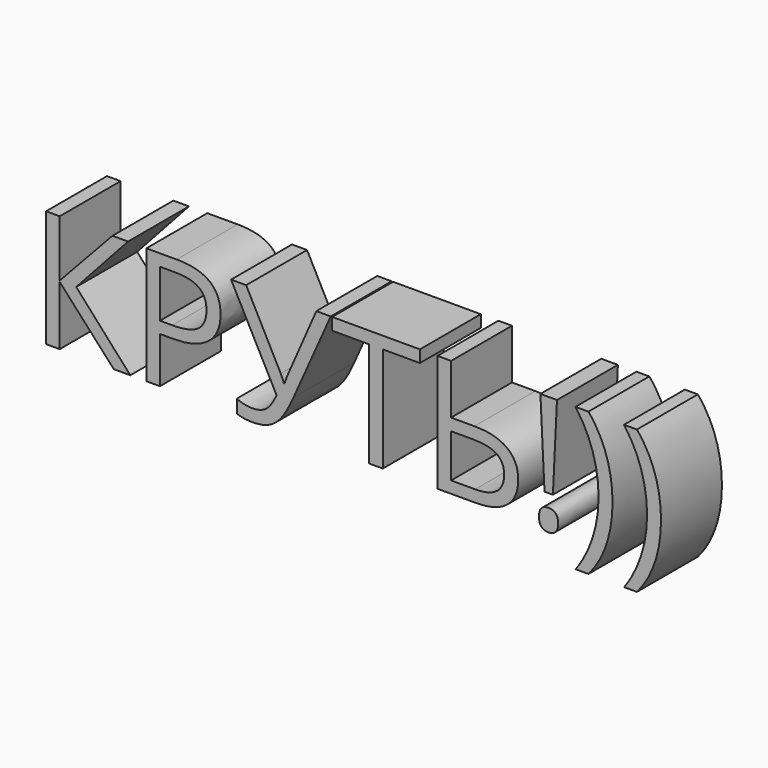
from build123d import *

# Parameters (mm, degrees)
F0_TEXT_SIZE = 53.8159886168
F1_DEPTH     = 25


# Not quite as in the source:
# - Text() gives the source's letters only with a copy of the font that has no kerning and outlines rounded to 1/6400 em; it was checked with that copy


with BuildPart() as f1:
    # F0 (on Front) → F1 (new body)
    with BuildSketch(Plane.XZ):
        with Locations((-64.8667886853, 39.7671833634)):
            Text('КРУТЬ!))', F0_TEXT_SIZE, font='Open Sans', text_align=(TextAlign.LEFT, TextAlign.BOTTOM))
    extrude(amount=F1_DEPTH)


solid = f1.part
